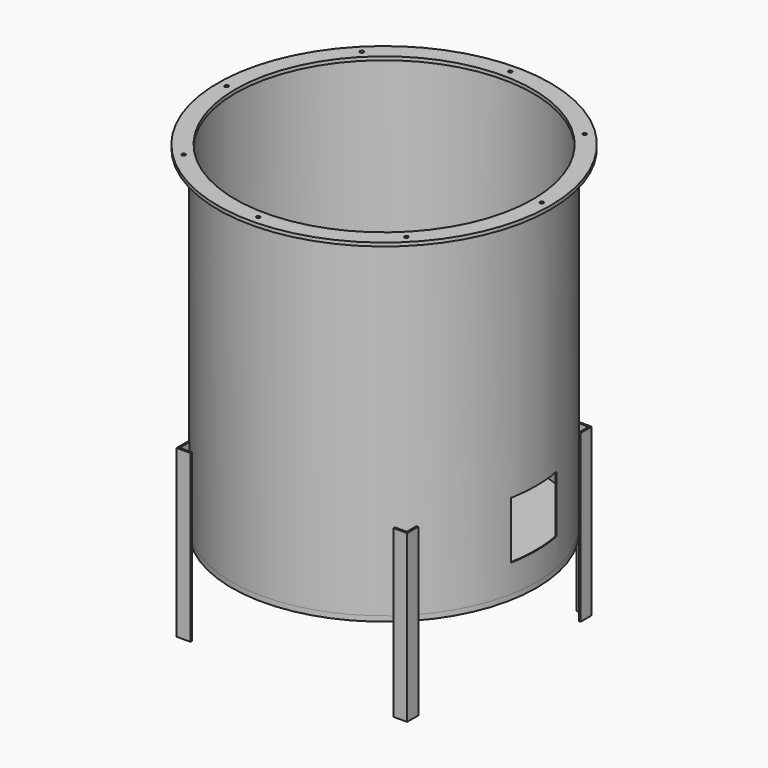
from build123d import *

# Parameters (mm, degrees)
F1_R            = 279.4
F2_DEPTH        = 9.525
F4_R            = 304.8
F4_R_2          = 273.05
F5_DEPTH        = 6.35
F6_R            = 279.4
F6_R_2          = 277.7744
F7_DEPTH        = 609.6
F8_D            = 6.7564
F8_COPIES_COUNT = 8
F11_DEPTH       = 304.8
F12_COUNT       = 4
F13_W           = 104.775
F13_H           = 104.775
F14_DEPTH       = 304.801


# Not quite as in the source:
# - a pattern or mirror of a feature is missing from the dataset's text; its kind, count and spacing are read off the source's solid


with BuildPart() as f2:
    # F1 (on offset) → F2 (new body)
    with BuildSketch(Plane.XY.offset(152.4)):
        Circle(F1_R)
    extrude(amount=F2_DEPTH)


with BuildPart() as f5:
    # F4 (on offset) → F5 (new body)
    with BuildSketch(Plane.XY.offset(771.525)):
        Circle(F4_R)
        Circle(F4_R_2, mode=Mode.SUBTRACT)
    extrude(amount=F5_DEPTH)

    # F8 (through all)
    with Locations(Plane(origin=(0, 0, 771.525), x_dir=(1, 0, 0), z_dir=(0, 0, -1))):
        with Locations((0, 288.925)):
            f8 = Hole(F8_D / 2)

    # F8_copies: F8 ×8 about axis
    f8_copies_axis = Axis((0, 0, 0), (0, 0, 1))
    for i in range(1, F8_COPIES_COUNT):
        add(f8.rotate(f8_copies_axis, i * 360 / F8_COPIES_COUNT), mode=Mode.SUBTRACT)


with BuildPart() as f7:
    # F6 (on face) → F7 (new body, through all)
    with BuildSketch(Plane.XY.offset(161.925)):
        Circle(F6_R)
        Circle(F6_R_2, mode=Mode.SUBTRACT)
    extrude(amount=F7_DEPTH)

    # F13 (on Right) → F14 (cut, through all)
    with BuildSketch(Plane.YZ):
        with Locations((0, 265.1125)):
            Rectangle(F13_W, F13_H)
    extrude(amount=F14_DEPTH, mode=Mode.SUBTRACT)


with BuildPart() as f11:
    # F10 (on Top) → F11 (new body)
    with BuildSketch(Plane.XY):
        Polygon((-208.3653639684, 208.3653639684), (-186.1403639684, 208.3653639684), (-186.1403639684, 211.5403639684), (-211.5403639684, 211.5403639684), (-211.5403639684, 186.1403639684), (-208.3653639684, 186.1403639684), align=None)
    extrude(amount=F11_DEPTH)


with BuildPart() as f12_1:
    # F12: instance of F11
    add(f11.part.rotate(Axis((0, 0, 467.6111340523), (0, 0, 1)), 1 * 360 / F12_COUNT))


with BuildPart() as f12_2:
    # F12: instance of F11
    add(f11.part.rotate(Axis((0, 0, 467.6111340523), (0, 0, 1)), 2 * 360 / F12_COUNT))


with BuildPart() as f12_3:
    # F12: instance of F11
    add(f11.part.rotate(Axis((0, 0, 467.6111340523), (0, 0, 1)), 3 * 360 / F12_COUNT))


solid = Compound([f2.part, f5.part, f7.part, f11.part, f12_1.part, f12_2.part, f12_3.part])
